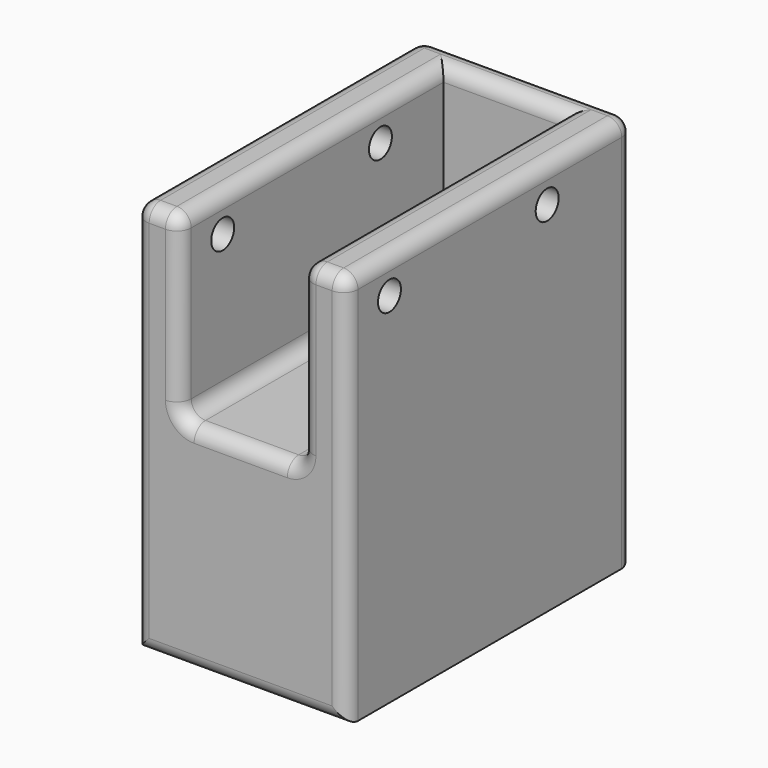
from build123d import *

# Parameters (mm, degrees)
F1_DEPTH  = 25
F2_DEPTH  = 5
F3_DEPTH  = 25
F4_R      = 2
F5_DEPTH  = 29.5357977842
F6_R      = 2
F7_DEPTH  = 29.5357977842
F8_R      = 1.99999
F9_R      = 1.5
F10_DEPTH = 15


# Not quite as in the source:
# - a fillet or chamfer is up to 0.001 mm smaller than in the source, because OpenCascade refuses the exact size
# - a feature names something its author has since deleted; it is built from what else it names


with BuildPart() as f1:
    # F0 (on Top) → F1 (new body)
    with BuildSketch(Plane.XY):
        Polygon((-8.5, -23.510635891), (-8.5, 0), (-8.5, 21), (8.5, 21), (8.5, 0), (8.5, -23.510635891), (8.5, -25), (14.7673988921, -25), (14.7673988921, -20.1723555878), (14.7673988921, -13.510635891), (14.7673988921, 25), (-14.7673988921, 25), (-14.7673988921, -20.1723555878), (-14.7673988921, -25), (-8.5, -25), align=None)
    extrude(amount=F1_DEPTH)

    # F0 (on Top) → F2 (join)
    with BuildSketch(Plane.XY):
        Polygon((-8.5, 21), (-8.5, 0), (-8.5, -23.510635891), (-8.5, -25), (8.5, -25), (8.5, -23.510635891), (8.5, 0), (8.5, 21), align=None)
        Polygon((-8.5, -23.510635891), (-8.5, 0), (-8.5, 21), (8.5, 21), (8.5, 0), (8.5, -23.510635891), (8.5, -25), (14.7673988921, -25), (14.7673988921, -20.1723555878), (14.7673988921, -13.510635891), (14.7673988921, 25), (-14.7673988921, 25), (-14.7673988921, -20.1723555878), (-14.7673988921, -25), (-8.5, -25), align=None)
    extrude(amount=-F2_DEPTH)

    # F3 (add): a face of the model
    f3_faces = [f1.faces().sort_by_distance(p)[0] for p in [
        (0, 0, -5),
    ]]
    extrude(f3_faces, amount=F3_DEPTH)

    # F4 (on face) → F5 (cut, through all)
    with BuildSketch(Plane.YZ.offset(14.7673988921)):
        with Locations((10, 20)):
            Circle(F4_R)
    extrude(amount=-F5_DEPTH, mode=Mode.SUBTRACT)

    # F6 (on face) → F7 (cut, through all)
    with BuildSketch(Plane.YZ.offset(14.7673988921)):
        with Locations((-17.510635891, 20)):
            Circle(F6_R)
    extrude(amount=-F7_DEPTH, mode=Mode.SUBTRACT)

    # F8 (radius 2 in the source; OpenCascade refuses exactly that, so slightly less here)
    f8_edges = [f1.edges().sort_by_distance(p)[0] for p in [
        (-11.633699, -25, 25),
        (-8.5, -2, 25),
        (0, 21, 25),
        (8.5, -2, 25),
        (11.633699, -25, 25),
        (14.767399, 0, 25),
        (0, 25, 25),
        (-14.767399, 0, 25),
        (-14.767399, 25, -2.5),
        (0, 25, -30),
        (14.767399, 25, -2.5),
        (-14.767399, -25, -2.5),
        (-8.5, -25, 12.5),
        (0, -25, 0),
        (8.5, -25, 12.5),
        (14.767399, -25, -2.5),
        (0, -25, -30),
        (-8.5, -2, 0),
        (0, 21, 0),
        (8.5, -2, 0),
    ]]
    fillet(f8_edges, radius=F8_R)

    # F9 (on face) → F10 (cut)
    with BuildSketch(Plane(origin=(0, 0, -30), x_dir=(1, 0, 0), z_dir=(0, 0, -1))):
        with Locations((9.2546826823, -4.7625)):
            Circle(F9_R)
        with Locations((1.0057907112, -9.525)):
            Circle(F9_R)
        with Locations((-7.2431012598, -4.7625)):
            Circle(F9_R)
        with Locations((-7.2431012598, 4.7625)):
            Circle(F9_R)
        with Locations((1.0057907112, 9.525)):
            Circle(F9_R)
        with Locations((9.2546826823, 4.7625)):
            Circle(F9_R)
    extrude(amount=-F10_DEPTH, mode=Mode.SUBTRACT)


solid = f1.part
